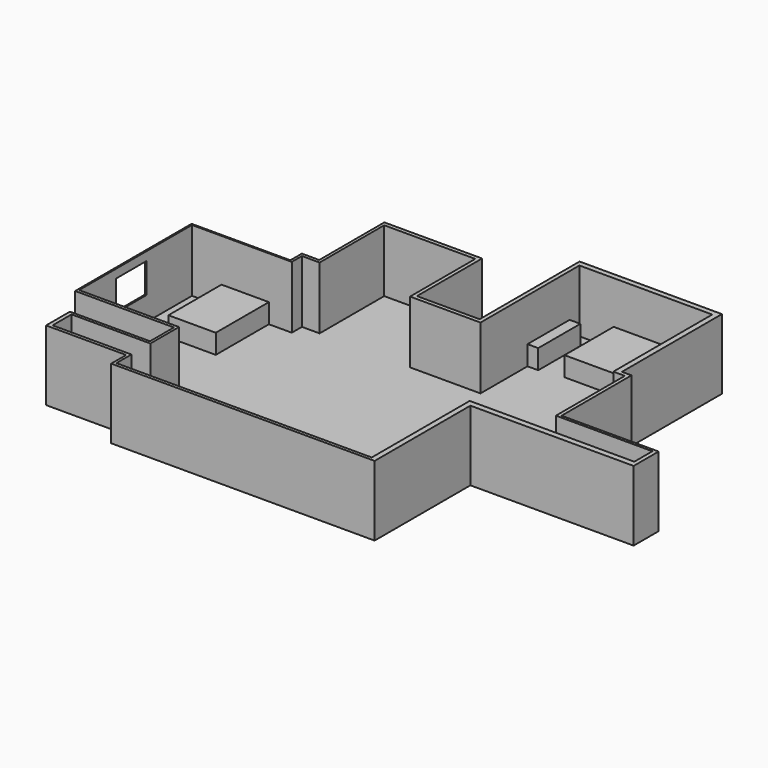
from build123d import *

# Parameters (mm, degrees)
F1_DEPTH  = 90
F3_DEPTH  = 80
F14_W     = 60.7640445232
F14_H     = 85.0984491408
F14_W_2   = 67.515194416
F14_H_2   = 10.8465999365
F15_DEPTH = 25
F16_W     = 49.2283031344
F16_H     = 38.4706258774
F17_DEPTH = 25
F18_W     = 81.171695143
F18_H     = 78.6929726601
F18_W_2   = 13.7816295028
F18_H_2   = 67.5387531519
F19_DEPTH = 25
F20_W     = 44.0124189481
F20_H     = 9.0348646045
F21_DEPTH = 70
F22_W     = 52.3186028004
F22_H     = 8.4803402424
F23_DEPTH = 25
F24_T     = -2.5


# Not quite as in the source:
# - a shell that OpenCascade refuses in one call is made with other operations: the cavity is built on its own and cut out
# - the program builds the solid bodies; features that only make, move or delete a surface that nothing else refers to are left out


with BuildPart() as f1:
    # F0 (on Top) → F1 (new body)
    with BuildSketch(Plane.XY):
        Polygon((0, -103.756165579), (61.2453594729, -103.756165579), (209.3763612108, -103.756165579), (209.3763612108, -63.756165579), (84.9471986294, -63.756165579), (84.9471986294, 48.3620613813), (72.6846382022, 48.3620613813), (72.6846382022, 208.6838036776), (-109.8914146423, 208.6838036776), (-109.8914146423, 48.3620613813), (-190.279379487, 48.3620613813), (-190.279379487, 152.8209894896), (-315.6301081181, 152.8209894896), (-315.6301081181, 48.3620613813), (-337.8433585167, 48.3620613813), (-337.8433585167, 29.8324227333), (-464.4817113876, 29.8324227333), (-464.4817113876, -156.8707674742), (-337.8433585167, -156.8707674742), (-337.8433585167, -195.1335072517), (-440.5674934387, -195.1335072517), (-440.5674934387, -233.3962619305), (-337.8433585167, -233.3962619305), (-337.8433585167, -257.3104500771), (0, -257.3104500771), align=None)
    extrude(amount=F1_DEPTH)

    # F2 (on face) → F3 (cut)
    with BuildSketch(Plane.XY.offset(90)):
        Polygon((-334.4984054565, 27.9887765646), (-462.5793099403, 27.9887765646), (-462.5793099403, -152.908667922), (-334.4984054565, -152.908667922), (-334.4984054565, -198.7856328487), (-435.5817735195, -198.7856328487), (-435.5817735195, -229.2267084122), (-334.4984054565, -229.2267084122), (-334.4984054565, -253.2849907875), (-6.9517553784, -253.2849907875), (-6.9517553784, -96.1697399616), (204.1718363762, -96.1697399616), (204.1718363762, -67.2016069293), (80.44359833, -67.2016069293), (80.44359833, 43.2700514793), (65.7140463591, 43.2700514793), (65.7140463591, 201.8582522869), (-104.6577990055, 201.8582522869), (-104.6577990055, 43.2700552046), (-194.9990689754, 43.2700552046), (-194.9990689754, 147.8498876095), (-311.8534982204, 147.8498876095), (-311.8534982204, 44.2520268261), (-334.4984054565, 44.2520268261), align=None)
    extrude(amount=-F3_DEPTH, mode=Mode.SUBTRACT)

    # F14 (on face) → F15 (join)
    with BuildSketch(Plane.XY.offset(10)):
        with Locations((-394.2892104387, -14.5604480058)):
            Rectangle(F14_W, F14_H)
        with Locations((-401.1757969856, -147.4853679538)):
            Rectangle(F14_W_2, F14_H_2)
    extrude(amount=F15_DEPTH)

    # F16 (on face) → F17 (cut)
    with BuildSketch(Plane.YZ.offset(-462.5793099403)):
        with Locations((-69.2342929542, 59.7355216742)):
            Rectangle(F16_W, F16_H)
    extrude(amount=-F17_DEPTH, mode=Mode.SUBTRACT)

    # F18 (on face) → F19 (join)
    with BuildSketch(Plane.XY.offset(10)):
        with Locations((-20.1654676348, 162.5117659569)):
            Rectangle(F18_W, F18_H)
        with Locations((-97.7669842541, 152.3723676801)):
            Rectangle(F18_W_2, F18_H_2)
    extrude(amount=F19_DEPTH)

    # F20 (on face) → F21 (join)
    with BuildSketch(Plane.XY.offset(10)):
        with Locations((31.1586786993, -91.6523076594)):
            Rectangle(F20_W, F20_H)
    extrude(amount=F21_DEPTH)

    # F22 (on face) → F23 (join)
    with BuildSketch(Plane.XY.offset(10)):
        with Locations((117.6677644253, -91.9295698404)):
            Rectangle(F22_W, F22_H)
    extrude(amount=F23_DEPTH)

    # F24: a shell. OpenCascade refuses it in one call, so the cavity is built on its own and cut out:
    # the body offset inwards by the wall thickness, plus a prism from it out through each open face.
    f24_core = offset(f1.part, amount=F24_T, kind=Kind.INTERSECTION, mode=Mode.PRIVATE)
    f24_exits = [f24_core.faces().sort_by_distance(p)[0] for p in [
        (31.158679, -89.634875, 42.5),
    ]]
    add(f24_core, mode=Mode.SUBTRACT)
    extrude(f24_exits, amount=-F24_T, mode=Mode.SUBTRACT)


solid = f1.part
